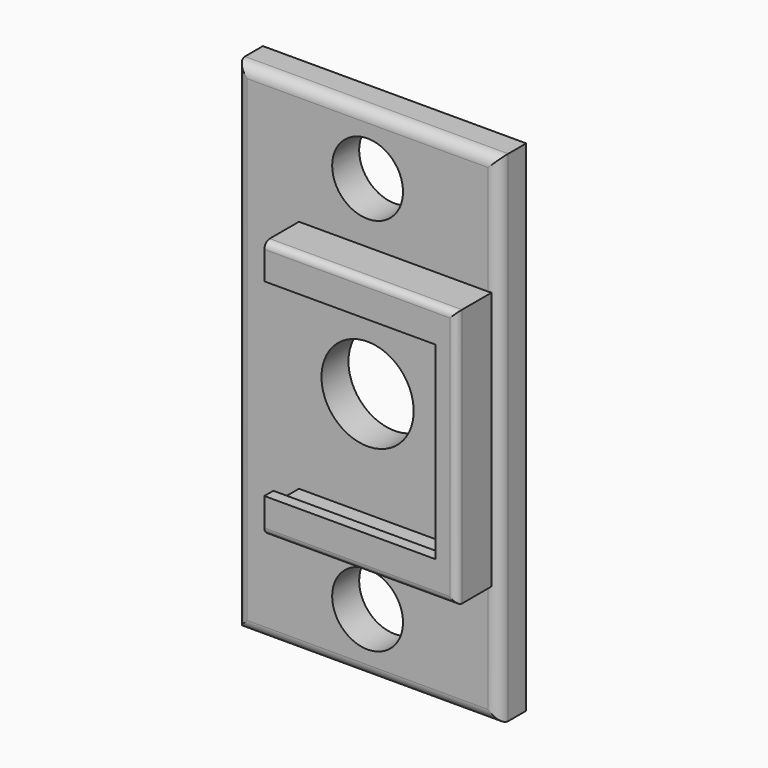
from build123d import *

# Parameters (mm, degrees)
F1_DEPTH      = 3
F2_DEPTH      = 6.85
F6_DEPTH      = 3
F3_W          = 16.2
F3_H          = 1
F7_DEPTH      = 1
F5_W          = 16.2
F5_H          = 1
F8_DEPTH      = 1
F4_W          = 1
F4_H          = 18.8
F9_DEPTH      = 1
F10_D         = 8.2
F0_W          = 23.4142135624
F0_H          = 44.4142135624
F11_DEPTH     = 3
F12_T1_DEPTH  = 28.4142135624
F12_T3_DEPTH  = 49.4142135624
F12_T8_DEPTH  = 49.4142135624
F12_T14_DEPTH = 49.4142135624
F12_T20_DEPTH = 49.4142135624
F12_T27_DEPTH = 49.4142135624
F12_T33_DEPTH = 49.4142135624
F13_R         = 0.6
F14_D         = 6.3


# Not quite as in the source:
# - a fillet or chamfer that OpenCascade refuses, or shapes differently, is made with other operations: its cross-section is extruded or revolved along the edge and cut away or added
# - a feature names something its author has since deleted; it is built from what else it names


with BuildPart() as f1:
    # F0 (on Front) → F1 (new body)
    with BuildSketch(Plane.XZ):
        Polygon((0.9, 2.1), (4.9, 2.1), (21.1, 2.1), (21.1, 20.9), (4.9, 20.9), (0.9, 20.9), align=None)
        Polygon((0, 23), (0, 0), (4.9, 0), (4.9, 2.1), (0.9, 2.1), (0.9, 20.9), (4.9, 20.9), (4.9, 23), align=None)
        Polygon((4.9, 2.1), (4.9, 0), (22, 0), (22, 23), (4.9, 23), (4.9, 20.9), (21.1, 20.9), (21.1, 2.1), align=None)
    extrude(amount=F1_DEPTH)

    # F0 (on Front) → F2 (join)
    with BuildSketch(Plane.XZ):
        Polygon((4.9, 2.1), (4.9, 0), (22, 0), (22, 23), (4.9, 23), (4.9, 20.9), (21.1, 20.9), (21.1, 2.1), align=None)
    extrude(amount=F2_DEPTH)

    # F0 (on Front) → F6 (join)
    with BuildSketch(Plane.XZ):
        Polygon((0, 23), (0, 0), (4.9, 0), (4.9, 2.1), (0.9, 2.1), (0.9, 20.9), (4.9, 20.9), (4.9, 23), align=None)
    extrude(amount=F6_DEPTH)

    # F3 (on face) → F7 (join)
    with BuildSketch(Plane(origin=(0, 0, 20.9), x_dir=(1, 0, 0), z_dir=(0, 0, -1))):
        with Locations((13, 6.35)):
            Rectangle(F3_W, F3_H)
    extrude(amount=F7_DEPTH)

    # F5 (on face) → F8 (join)
    with BuildSketch(Plane.XY.offset(2.1)):
        with Locations((13, -6.35)):
            Rectangle(F5_W, F5_H)
    extrude(amount=F8_DEPTH)

    # F4 (on face) → F9 (join)
    with BuildSketch(Plane(origin=(21.1, 0, 0), x_dir=(0, -1, 0), z_dir=(-1, 0, 0))):
        with Locations((6.35, 11.5)):
            Rectangle(F4_W, F4_H)
    extrude(amount=F9_DEPTH)

    # F10 (through all)
    with Locations(Plane(origin=(0, 0, 0), x_dir=(1, 0, 0), z_dir=(0, 1, 0))):
        with Locations((11, -11.5)):
            Hole(F10_D / 2)

    # F0 (on Front) → F11 (join)
    with BuildSketch(Plane.XZ):
        with Locations((11, 11.5)):
            Rectangle(F0_W, F0_H)
        Polygon((4.9, 0), (0, 0), (0, 23), (4.9, 23), (22, 23), (22, 0), align=None, mode=Mode.SUBTRACT)
    extrude(amount=F11_DEPTH)

    # F12: fillet of radius 1 on 4 edges, made by hand

    # F12_s2 → F12_t1 (cut)
    with BuildSketch(Plane.YZ.offset(-3.2071067812)):
        with BuildLine():
            ThreePointArc((-3, -9.7071067812), (-2.7071067812, -10.4142135624), (-2, -10.7071067812))
            Line((-2, -10.7071067812), (-3, -10.7071067812))
            Line((-3, -10.7071067812), (-3, -9.7071067812))
        make_face()
        with BuildLine():
            ThreePointArc((-3, 32.7071067812), (-2.7071067812, 33.4142135624), (-2, 33.7071067812))
            Line((-2, 33.7071067812), (-3, 33.7071067812))
            Line((-3, 33.7071067812), (-3, 32.7071067812))
        make_face()
    extrude(amount=F12_T1_DEPTH, mode=Mode.SUBTRACT)

    # F12_s4 → F12_t3 (cut)
    with BuildSketch(Plane.XY.offset(-13.2071067812)):
        with BuildLine():
            ThreePointArc((0.2928932188, -3), (-0.4142135624, -2.7071067812), (-0.7071067812, -2))
            Line((-0.7071067812, -2), (-0.7071067812, -3))
            Line((-0.7071067812, -3), (0.2928932188, -3))
        make_face()
    extrude(amount=F12_T3_DEPTH, mode=Mode.SUBTRACT)


with BuildPart() as f12_tool6:
    # F12_s7 → F12_t8 (new body)
    with BuildSketch(Plane.XY.offset(-13.2071067812)):
        with BuildLine():
            ThreePointArc((21.7071067812, -3), (22.4142135624, -2.7071067812), (22.7071067812, -2))
            Line((22.7071067812, -2), (22.7071067812, -3))
            Line((22.7071067812, -3), (21.7071067812, -3))
        make_face()
    extrude(amount=F12_T8_DEPTH)

    split(bisect_by=Plane.XY, keep=Keep.BOTTOM)

    split(bisect_by=Plane.YZ.offset(22), keep=Keep.BOTTOM)


with BuildPart() as f1_1:
    add(f1.part)

    # F12_t5: cut F12_tool6
    add(f12_tool6.part, mode=Mode.SUBTRACT)


with BuildPart() as f12_tool12:
    # F12_s13 → F12_t14 (new body)
    with BuildSketch(Plane.XY.offset(-13.2071067812)):
        with BuildLine():
            ThreePointArc((21.7071067812, -3), (22.4142135624, -2.7071067812), (22.7071067812, -2))
            Line((22.7071067812, -2), (22.7071067812, -3))
            Line((22.7071067812, -3), (21.7071067812, -3))
        make_face()
    extrude(amount=F12_T14_DEPTH)

    split(bisect_by=Plane.XY, keep=Keep.BOTTOM)

    split(bisect_by=Plane.YZ.offset(22), keep=Keep.TOP)


with BuildPart() as f1_2:
    add(f1_1.part)

    # F12_t11: cut F12_tool12
    add(f12_tool12.part, mode=Mode.SUBTRACT)


with BuildPart() as f12_tool18:
    # F12_s19 → F12_t20 (new body)
    with BuildSketch(Plane.XY.offset(-13.2071067812)):
        with BuildLine():
            ThreePointArc((21.7071067812, -3), (22.4142135624, -2.7071067812), (22.7071067812, -2))
            Line((22.7071067812, -2), (22.7071067812, -3))
            Line((22.7071067812, -3), (21.7071067812, -3))
        make_face()
    extrude(amount=F12_T20_DEPTH)

    split(bisect_by=Plane.XY.offset(23), keep=Keep.BOTTOM)

    split(bisect_by=Plane.XY, keep=Keep.TOP)

    split(bisect_by=Plane.YZ.offset(22), keep=Keep.TOP)


with BuildPart() as f1_3:
    add(f1_2.part)

    # F12_t17: cut F12_tool18
    add(f12_tool18.part, mode=Mode.SUBTRACT)


with BuildPart() as f12_tool25:
    # F12_s26 → F12_t27 (new body)
    with BuildSketch(Plane.XY.offset(-13.2071067812)):
        with BuildLine():
            ThreePointArc((21.7071067812, -3), (22.4142135624, -2.7071067812), (22.7071067812, -2))
            Line((22.7071067812, -2), (22.7071067812, -3))
            Line((22.7071067812, -3), (21.7071067812, -3))
        make_face()
    extrude(amount=F12_T27_DEPTH)

    split(bisect_by=Plane.XY.offset(23), keep=Keep.TOP)

    split(bisect_by=Plane.YZ.offset(22), keep=Keep.BOTTOM)


with BuildPart() as f1_4:
    add(f1_3.part)

    # F12_t24: cut F12_tool25
    add(f12_tool25.part, mode=Mode.SUBTRACT)


with BuildPart() as f12_tool31:
    # F12_s32 → F12_t33 (new body)
    with BuildSketch(Plane.XY.offset(-13.2071067812)):
        with BuildLine():
            ThreePointArc((21.7071067812, -3), (22.4142135624, -2.7071067812), (22.7071067812, -2))
            Line((22.7071067812, -2), (22.7071067812, -3))
            Line((22.7071067812, -3), (21.7071067812, -3))
        make_face()
    extrude(amount=F12_T33_DEPTH)

    split(bisect_by=Plane.XY.offset(23), keep=Keep.TOP)

    split(bisect_by=Plane.YZ.offset(22), keep=Keep.TOP)


with BuildPart() as f1_5:
    add(f1_4.part)

    # F12_t30: cut F12_tool31
    add(f12_tool31.part, mode=Mode.SUBTRACT)

    # F13
    f13_edges = [f1_5.edges().sort_by_distance(p)[0] for p in [
        (22, -6.85, 11.5),
        (13.45, -6.85, 0),
        (13.45, -6.85, 23),
    ]]
    fillet(f13_edges, radius=F13_R)

    # F14 (through all)
    with Locations(Plane(origin=(0, 0, 0), x_dir=(1, 0, 0), z_dir=(0, 1, 0))):
        with Locations((11, -28.3535533906), (11, 5.3535533906)):
            Hole(F14_D / 2)


solid = f1_5.part
